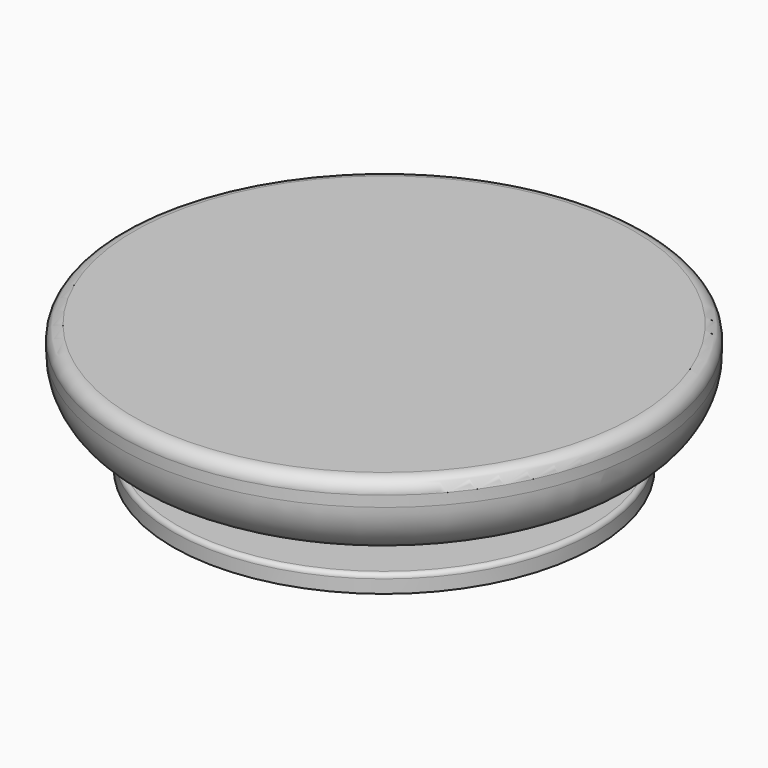
from build123d import *

# Parameters (mm, degrees)
F0_R      = 48
F1_DEPTH  = 4
F2_R      = 1
F3_R      = 35.5
F4_DEPTH  = 3.5
F5_SIZE   = 3
F6_R      = 35.5
F6_R_2    = 32.5
F7_DEPTH  = 3.5
F8_SIZE   = 2.99999
F9_R      = 60
F9_R_2    = 47.0001739343
F9_R_3    = 35.5
F10_DEPTH = 18
F11_R     = 12.5539105243
F12_R     = 3


# Not quite as in the source:
# - a fillet or chamfer is up to 0.001 mm smaller than in the source, because OpenCascade refuses the exact size


with BuildPart() as f1:
    # F0 (on Top) → F1 (new body)
    with BuildSketch(Plane.XY):
        Circle(F0_R)
    extrude(amount=F1_DEPTH)

    # F2
    f2_edges = [f1.edges().sort_by_distance(p)[0] for p in [
        (-48, 0, 4),
    ]]
    fillet(f2_edges, radius=F2_R)

    # F3 (on face) → F4 (join)
    with BuildSketch(Plane.XY.offset(4)):
        Circle(F3_R)
    extrude(amount=F4_DEPTH)

    # F5
    f5_edges = [f1.edges().sort_by_distance(p)[0] for p in [
        (-35.5, 0, 7.5),
    ]]
    chamfer(f5_edges, length=F5_SIZE)

    # F6 (on face) → F7 (join)
    with BuildSketch(Plane.XY.offset(7.5)):
        Circle(F6_R)
        Circle(F6_R_2, mode=Mode.SUBTRACT)
        Circle(F6_R_2)
    extrude(amount=F7_DEPTH)

    # F8 (size 3 in the source; OpenCascade refuses exactly that, so slightly less here)
    f8_edges = [f1.edges().sort_by_distance(p)[0] for p in [
        (-35.5, 0, 7.5),
    ]]
    chamfer(f8_edges, length=F8_SIZE)

    # F9 (on face) → F10 (join)
    with BuildSketch(Plane.XY.offset(11)):
        Circle(F9_R)
        Circle(F9_R_2, mode=Mode.SUBTRACT)
        Circle(F9_R_2)
        Circle(F9_R_3, mode=Mode.SUBTRACT)
        Circle(F9_R_3)
    extrude(amount=F10_DEPTH)

    # F11
    f11_edges = [f1.edges().sort_by_distance(p)[0] for p in [
        (-60, 0, 11),
    ]]
    fillet(f11_edges, radius=F11_R)

    # F12
    f12_edges = [f1.edges().sort_by_distance(p)[0] for p in [
        (-60, 0, 29),
    ]]
    fillet(f12_edges, radius=F12_R)


solid = f1.part
